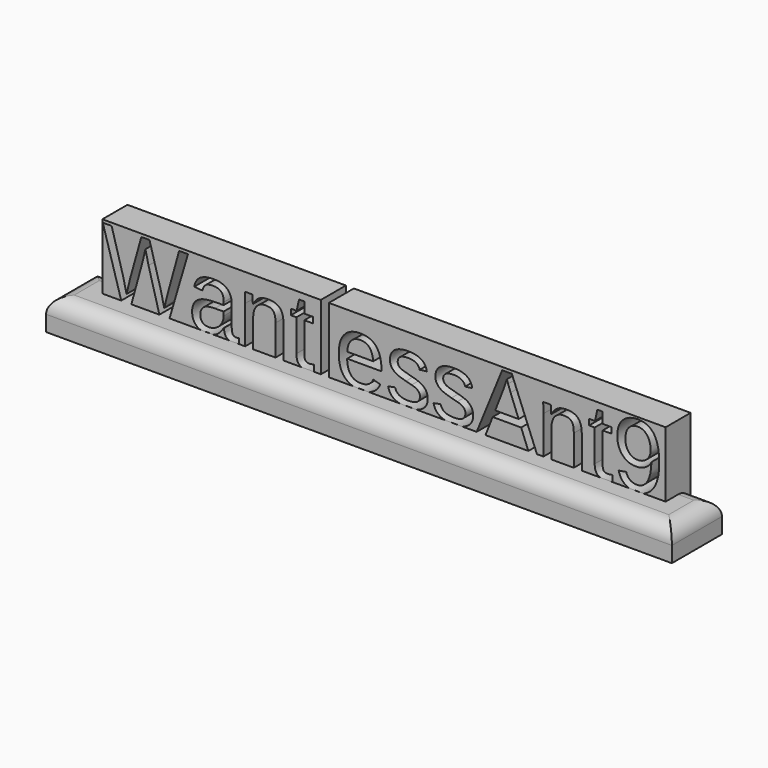
from build123d import *

# Parameters (mm, degrees)
F1_DEPTH     = 10
F2_W         = 180
F2_H         = 10
F3_DEPTH     = 20.93
F5_DEPTH     = 10
F6_R         = 5
F4_TEXT_SIZE = 29.0732889158
F8_DEPTH     = 10


# Not quite as in the source:
# - Text() gives the source's letters only with a copy of the font that has no kerning and outlines rounded to 1/6400 em; it was checked with that copy


with BuildPart() as f1:
    # F0 (on Top) → F1 (new body)
    with BuildSketch(Plane.XY):
        Polygon((100, 10), (0, 10), (-100, 10), (-100, -20), (100, -20), align=None)
    extrude(amount=F1_DEPTH)

    # F2 (on face) → F3 (join)
    with BuildSketch(Plane.XY.offset(10)):
        with Locations((0, 5)):
            Rectangle(F2_W, F2_H)
    extrude(amount=F3_DEPTH)

    # F5 (cut): a face of the model
    f5_faces = [f1.faces().sort_by_distance(p)[0] for p in [
        (0, -20, 5),
    ]]
    extrude(f5_faces, amount=-F5_DEPTH, mode=Mode.SUBTRACT)

    # F6
    f6_edges = [f1.edges().sort_by_distance(p)[0] for p in [
        (-100, 0, 10),
        (0, -10, 10),
        (100, 0, 10),
        (95, 10, 10),
        (-95, 10, 10),
    ]]
    fillet(f6_edges, radius=F6_R)


with BuildPart() as f7_1:
    # F7: copy of F1
    add(f1.part)


with BuildPart() as f8_tool:
    # F4 (on face) → F8 (new body)
    with BuildSketch(Plane.XZ):
        with Locations((-90, 10)):
            Text('WantlessAnt9', F4_TEXT_SIZE, font='Arimo', text_align=(TextAlign.LEFT, TextAlign.BOTTOM))
    extrude(amount=-F8_DEPTH)


with BuildPart() as f1_1:
    add(f1.part)

    # F8: cut by f8_tool
    add(f8_tool.part, mode=Mode.SUBTRACT)


with BuildPart() as f7_1_1:
    add(f7_1.part)

    # F8: cut by f8_tool
    add(f8_tool.part, mode=Mode.SUBTRACT)


solid = Compound([f1_1.part, f7_1_1.part])
